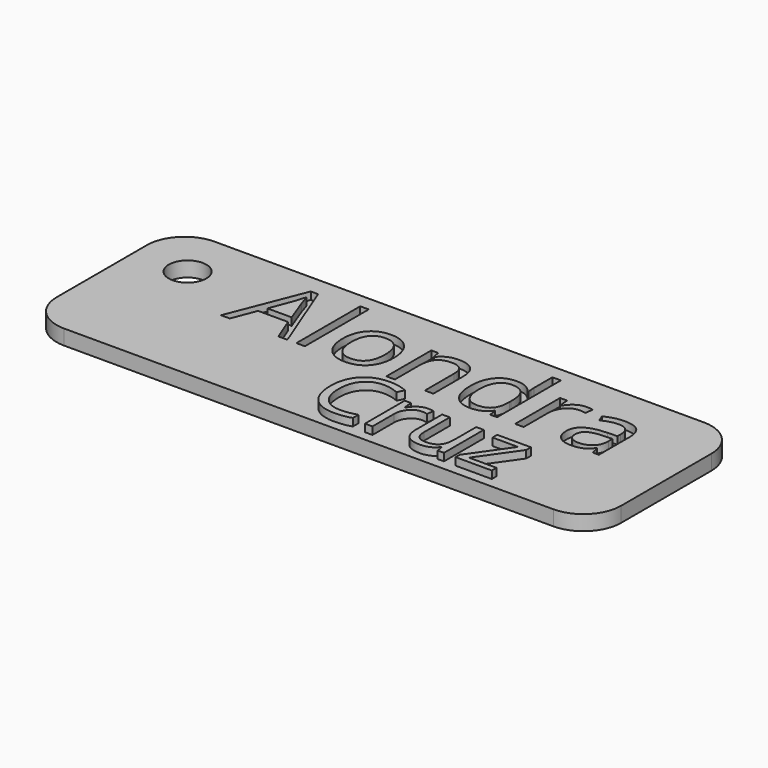
from build123d import *

# Parameters (mm, degrees)
F1_DEPTH     = 2
F3_D         = 5
F4_TEXT_SIZE = 13.9458117903
F5_DEPTH     = 1
F6_TEXT_SIZE = 12.3520029269
F7_DEPTH     = 1


# Not quite as in the source:
# - Text() gives the source's letters only with a copy of the font that has no kerning and outlines rounded to 1/6400 em; it was checked with that copy


with BuildPart() as f1:
    # F0 (on Top) → F1 (new body)
    with BuildSketch(Plane.XY):
        with BuildLine():
            Line((32.5, 12.5), (-32.5, 12.5))
            ThreePointArc((-32.5, 12.5), (-36.0355339059, 11.0355339059), (-37.5, 7.5))
            Line((-37.5, 7.5), (-37.5, -7.5))
            ThreePointArc((-37.5, -7.5), (-36.0355339059, -11.0355339059), (-32.5, -12.5))
            Line((-32.5, -12.5), (32.5, -12.5))
            ThreePointArc((32.5, -12.5), (36.0355339059, -11.0355339059), (37.5, -7.5))
            Line((37.5, -7.5), (37.5, 7.5))
            ThreePointArc((37.5, 7.5), (36.0355339059, 11.0355339059), (32.5, 12.5))
        make_face()
    extrude(amount=F1_DEPTH)

    # F3 (through all)
    with Locations(Plane.XY.offset(2)):
        with Locations((-30.5, 5.5)):
            Hole(F3_D / 2)

    # F4 (on face) → F5 (cut)
    with BuildSketch(Plane.XY.offset(2)):
        with Locations((-21.6598380357, 0)):
            Text('Alondra', F4_TEXT_SIZE, font='Open Sans', text_align=(TextAlign.LEFT, TextAlign.BOTTOM))
    extrude(amount=-F5_DEPTH, mode=Mode.SUBTRACT)

    # F6 (on face) → F7 (join)
    with BuildSketch(Plane.XY.offset(2)):
        with Locations((-2.4385238066, -11.1885247752)):
            Text('Cruz', F6_TEXT_SIZE, font='Open Sans', text_align=(TextAlign.LEFT, TextAlign.BOTTOM))
    extrude(amount=F7_DEPTH)


solid = f1.part
